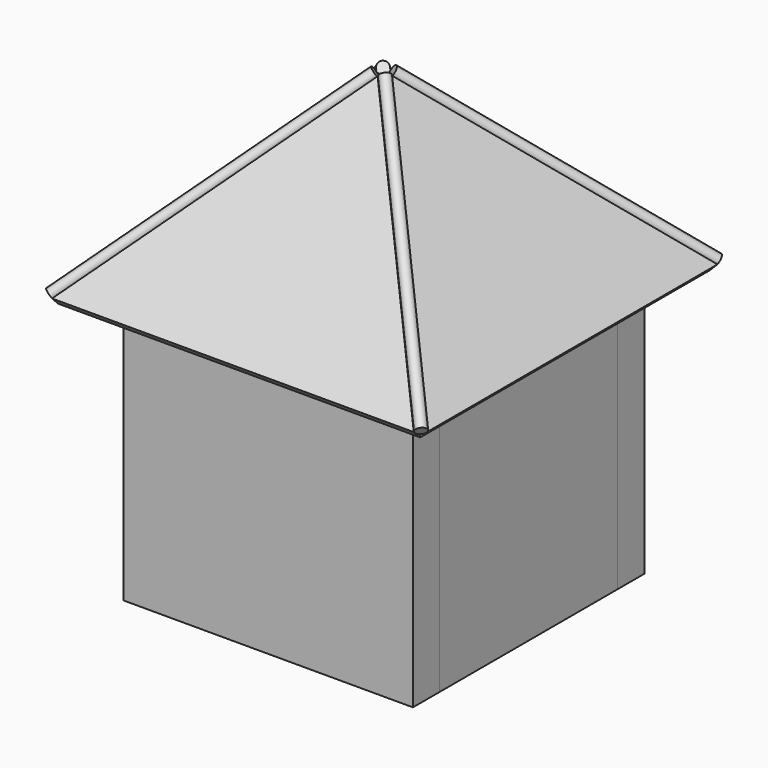
from build123d import *

# Parameters (mm, degrees)
F2_DEPTH  = 19.05
F4_W      = 127
F4_H      = 190.5
F5_DEPTH  = 19.05
F6_SIZE2  = 19.04999
F6_SIZE   = 19.04999
F8_W      = 127
F8_H      = 190.5
F9_DEPTH  = 19.05
F10_SIZE2 = 19.04999
F10_SIZE  = 19.04999
F13_DEPTH = 19.05
F14_SIZE2 = 19.04999
F14_SIZE  = 19.04999
F17_DEPTH = 19.05
F18_SIZE2 = 19.04999
F18_SIZE  = 19.04999
F21_DEPTH = 6.35
F25_DEPTH = 6.35
F28_R     = 3.175
F29_DEPTH = 178.562
F30_COUNT = 4
F30_ANGLE = 270


# Not quite as in the source:
# - a fillet or chamfer is up to 0.001 mm smaller than in the source, because OpenCascade refuses the exact size


with BuildPart() as f2:
    # F1 (on Top) → F2 (new body)
    with BuildSketch(Plane.XY):
        Polygon((-50.8, -63.5), (50.8, -63.5), (63.5, -50.8), (63.5, 50.8), (50.8, 63.5), (-50.8, 63.5), (-63.5, 50.8), (-63.5, -50.8), align=None)
    extrude(amount=F2_DEPTH)


with BuildPart() as f5:
    # F4 (on offset) → F5 (new body)
    with BuildSketch(Plane.YZ.offset(63.5508)):
        with Locations((0, 95.25)):
            Rectangle(F4_W, F4_H)
    extrude(amount=F5_DEPTH)

    # F6 (size 19.05 and 19.05 in the source; OpenCascade refuses exactly that, so slightly less here)
    f6_edges = [f5.edges().sort_by_distance(p)[0] for p in [
        (82.6008, 0, 190.5),
    ]]
    chamfer(f6_edges, length=F6_SIZE, length2=F6_SIZE2)


with BuildPart() as f9:
    # F8 (on offset) → F9 (new body)
    with BuildSketch(Plane.YZ.offset(-63.5508)):
        with Locations((0, 95.25)):
            Rectangle(F8_W, F8_H)
    extrude(amount=-F9_DEPTH)

    # F10 (size 19.05 and 19.05 in the source; OpenCascade refuses exactly that, so slightly less here)
    f10_edges = [f9.edges().sort_by_distance(p)[0] for p in [
        (-82.6008, 0, 190.5),
    ]]
    chamfer(f10_edges, length=F10_SIZE, length2=F10_SIZE2)


with BuildPart() as f13:
    # F12 (on offset) → F13 (new body)
    with BuildSketch(Plane.XZ.offset(-63.5508)):
        Polygon((-82.6008, 0), (82.6008, 0), (82.6008, 171.45), (63.5508, 190.5), (-63.5508, 190.5), (-82.6008, 171.45), align=None)
    extrude(amount=-F13_DEPTH)

    # F14 (size 19.05 and 19.05 in the source; OpenCascade refuses exactly that, so slightly less here)
    f14_edges = [f13.edges().sort_by_distance(p)[0] for p in [
        (0, 82.6008, 190.5),
    ]]
    chamfer(f14_edges, length=F14_SIZE, length2=F14_SIZE2)


with BuildPart() as f17:
    # F16 (on offset) → F17 (new body)
    with BuildSketch(Plane.XZ.offset(63.5508)):
        Polygon((-82.6008, 171.45), (-82.6008, 0), (82.6008, 0), (82.6008, 171.45), (63.5508, 190.5), (-63.5508, 190.5), align=None)
    extrude(amount=F17_DEPTH)

    # F18 (size 19.05 and 19.05 in the source; OpenCascade refuses exactly that, so slightly less here)
    f18_edges = [f17.edges().sort_by_distance(p)[0] for p in [
        (0, -82.6008, 190.5),
    ]]
    chamfer(f18_edges, length=F18_SIZE, length2=F18_SIZE2)


with BuildPart() as f21:
    # F20 (on offset) → F21 (new body)
    with BuildSketch(Plane(origin=(127.0613210245, 0, 127.0613210245), x_dir=(0.7071067812, 0, -0.7071067812), z_dir=(0.7071067812, 0, 0.7071067812))):
        Polygon((-33.5910434459, 103.2729453923), (-179.6410434459, 0), (-33.5910434459, -103.2729453923), align=None)
    extrude(amount=F21_DEPTH)


with BuildPart() as f22_1:
    # F22: instance of F21
    add(f21.part.mirror(Plane.YZ))


with BuildPart() as f25:
    # F24 (on offset) → F25 (new body)
    with BuildSketch(Plane(origin=(0, -127.097242049, 127.097242049), x_dir=(1, 0, 0), z_dir=(0, -0.7071067812, 0.7071067812))):
        Polygon((0, 179.6410434459), (-103.2729453923, 33.5910434459), (103.2729453923, 33.5910434459), align=None)
    extrude(amount=F25_DEPTH)


with BuildPart() as f26_1:
    # F26: instance of F25
    add(f25.part.mirror(Plane.XZ))


with BuildPart() as f29:
    # F28 (on 3pt) → F29 (new body)
    with BuildSketch(Plane(origin=(18.5893453923, -18.5893453923, -18.5893453923), x_dir=(0.8164965809, 0.4082482905, 0.4082482905), z_dir=(0.5773502692, -0.5773502692, -0.5773502692))):
        with Locations((106.890804791, 185.1403047599)):
            Circle(F28_R)
    extrude(amount=-F29_DEPTH)


with BuildPart() as f30_1:
    # F30: instance of F29
    add(f29.part.rotate(Axis((0, 0, 21.357871592), (0, 0, 1)), 1 * F30_ANGLE / (F30_COUNT - 1)))


with BuildPart() as f30_2:
    # F30: instance of F29
    add(f29.part.rotate(Axis((0, 0, 21.357871592), (0, 0, 1)), 2 * F30_ANGLE / (F30_COUNT - 1)))


with BuildPart() as f30_3:
    # F30: instance of F29
    add(f29.part.rotate(Axis((0, 0, 21.357871592), (0, 0, 1)), 3 * F30_ANGLE / (F30_COUNT - 1)))


solid = Compound([f2.part, f5.part, f9.part, f13.part, f17.part, f21.part, f22_1.part, f25.part, f26_1.part, f29.part, f30_1.part, f30_2.part, f30_3.part])
